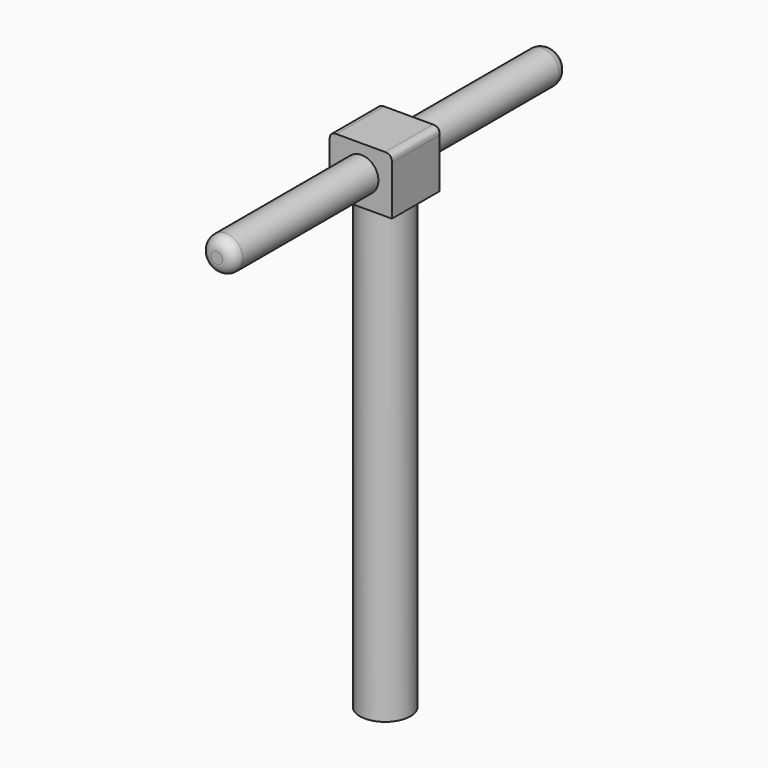
from build123d import *

# Parameters (mm, degrees)
F0_R        = 11.1966523668
F1_DEPTH    = 200
F2_W        = 27.5912405923
F2_H        = 26.4416076243
F3_DEPTH    = 25
F5_R        = 7.5599777125
F6_DEPTH    = 80
F4_R        = 7.5148466093
F7_DEPTH    = 80
F8_T1_DEPTH = 41.4416076243
F9_R        = 5
F10_R       = 5


# Not quite as in the source:
# - a fillet or chamfer that OpenCascade refuses, or shapes differently, is made with other operations: its cross-section is extruded or revolved along the edge and cut away or added
# - a feature names something its author has since deleted; it is built from what else it names


with BuildPart() as f1:
    # F0 (on Top) → F1 (new body)
    with BuildSketch(Plane.XY):
        Circle(F0_R)
    extrude(amount=F1_DEPTH)

    # F2 (on face) → F3 (join)
    with BuildSketch(Plane.XY.offset(200)):
        with Locations((-0.2874094062, 0.0958032906)):
            Rectangle(F2_W, F2_H)
    extrude(amount=F3_DEPTH)

    # F5 (on face) → F6 (join)
    with BuildSketch(Plane(origin=(0, 13.3166071028, 0), x_dir=(-1, 0, 0), z_dir=(0, 1, 0))):
        with Locations((1.2183021754, 212.9181474447)):
            Circle(F5_R)
    extrude(amount=F6_DEPTH)

    # F4 (on face) → F7 (join)
    with BuildSketch(Plane.XZ.offset(13.1250005215)):
        with Locations((0, 212.9505872726)):
            Circle(F4_R)
    extrude(amount=F7_DEPTH)

    # F8: fillet of radius 3 on 2 edges, made by hand

    # F8_s2 → F8_t1 (cut)
    with BuildSketch(Plane.XZ.offset(-20.8166071028)):
        with BuildLine():
            add(Edge.make_bspline(
                [(13.50821089, 222), (13.50821089, 225), (10.50821089, 225)],
                knots=[0, 0, 0, 1, 1, 1], degree=2, weights=[1, 1, 1]))
            Line((10.50821089, 225), (13.50821089, 225))
            Line((13.50821089, 225), (13.50821089, 222))
        make_face()
        with BuildLine():
            add(Edge.make_bspline(
                [(-11.0830297023, 225), (-14.0830297023, 225), (-14.0830297023, 222)],
                knots=[0, 0, 0, 1, 1, 1], degree=2, weights=[1, 1, 1]))
            Line((-14.0830297023, 222), (-14.0830297023, 225))
            Line((-14.0830297023, 225), (-11.0830297023, 225))
        make_face()
    extrude(amount=F8_T1_DEPTH, mode=Mode.SUBTRACT)

    # F9
    f9_edges = [f1.edges().sort_by_distance(p)[0] for p in [
        (6.341676, 93.316607, 212.918147),
    ]]
    fillet(f9_edges, radius=F9_R)

    # F10
    f10_edges = [f1.edges().sort_by_distance(p)[0] for p in [
        (-7.514847, -93.125001, 212.950587),
    ]]
    fillet(f10_edges, radius=F10_R)


solid = f1.part
